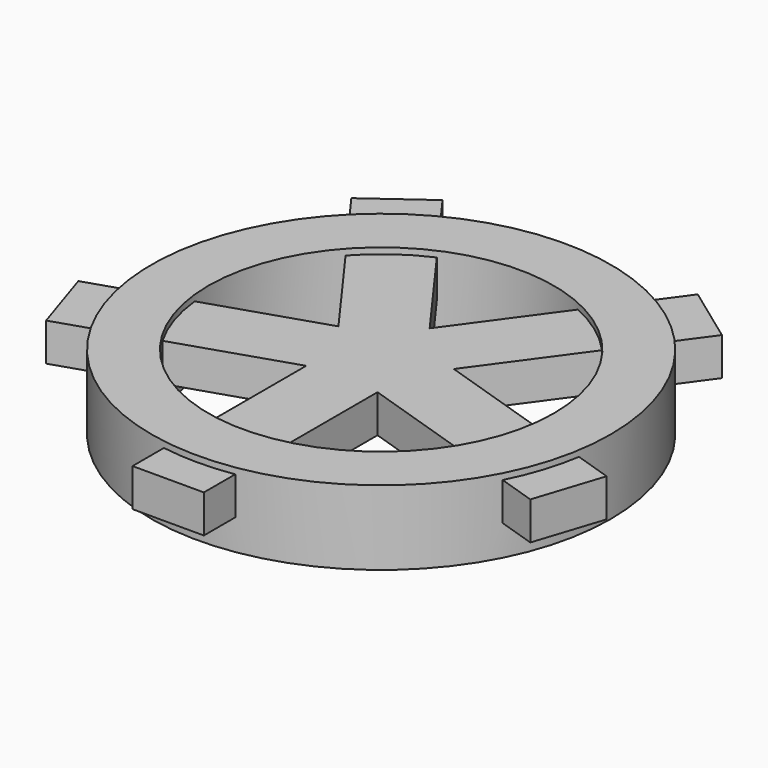
from build123d import *

# Parameters (mm, degrees)
F0_R            = 78.299536584
F0_R_2          = 58.8964149972
F1_DEPTH        = 25.4
F2_W            = 24.3125222623
F2_H            = 12.9293575883
F3_DEPTH        = 90.7285287976
F3_COPIES_COUNT = 5


# Not quite as in the source:
# - a pattern or mirror of a feature is missing from the dataset's text; its kind, count and spacing are read off the source's solid


with BuildPart() as f1:
    # F0 (on Top) → F1 (new body)
    with BuildSketch(Plane.XY):
        Circle(F0_R)
        Circle(F0_R_2, mode=Mode.SUBTRACT)
    extrude(amount=F1_DEPTH)

    # F2 (on Front) → F3 (join)
    with BuildSketch(Plane.XZ):
        with Locations((0, 16.8866589665)):
            Rectangle(F2_W, F2_H)
    f3 = extrude(amount=F3_DEPTH)

    # F3_copies: F3 ×5 about axis
    f3_copies_axis = Axis((0, 0, 0), (0, 0, 1))
    for i in range(1, F3_COPIES_COUNT):
        add(f3.rotate(f3_copies_axis, i * 360 / F3_COPIES_COUNT))


solid = f1.part
